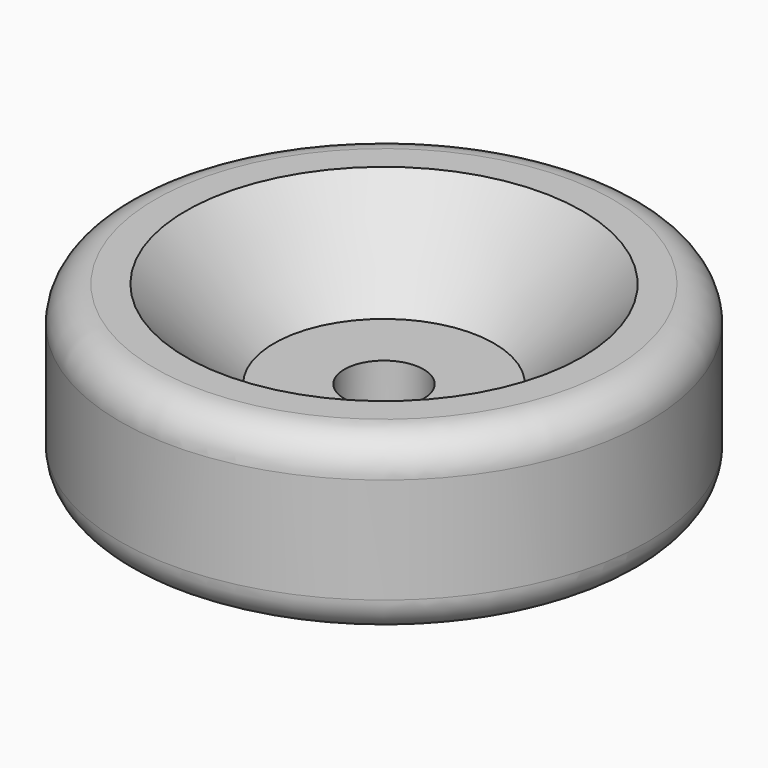
from build123d import *

# Parameters (mm, degrees)
F0_R     = 15
F0_R_2   = 11
F0_R_3   = 4.25
F1_DEPTH = 10
F2_R     = 2
F0_R_4   = 2.25
F3_DEPTH = 5


# Not quite as in the source:
# - a fillet or chamfer that OpenCascade refuses, or shapes differently, is made with other operations: its cross-section is extruded or revolved along the edge and cut away or added


with BuildPart() as f1:
    # F0 (on Top) → F1 (new body)
    with BuildSketch(Plane.XY):
        Circle(F0_R)
        Circle(F0_R_2, mode=Mode.SUBTRACT)
        Circle(F0_R_2)
        Circle(F0_R_3, mode=Mode.SUBTRACT)
    extrude(amount=F1_DEPTH)

    # F2
    f2_edges = [f1.edges().sort_by_distance(p)[0] for p in [
        (-15, 0, 10),
        (15, 0, 5),
        (-15, 0, 0),
    ]]
    fillet(f2_edges, radius=F2_R)

    # F0 (on Top) → F3 (join)
    with BuildSketch(Plane.XY):
        Circle(F0_R_3)
        Circle(F0_R_4, mode=Mode.SUBTRACT)
    extrude(amount=F3_DEPTH)

    # F4: chamfer of 7 on 1 edges, made by hand


with BuildPart() as f4_tool2:
    # F4_s3 → F4_t4 (revolve)
    with BuildSketch(Plane.XZ):
        Polygon((11.25, 10), (4.25, 3), (4.25, 10), align=None)
    revolve(axis=Axis((0, 0, 10), (0, 0, 1)))

    split(bisect_by=Plane.XY.offset(5), keep=Keep.TOP)


with BuildPart() as f1_1:
    add(f1.part)

    # F4_t1: cut F4_tool2
    add(f4_tool2.part, mode=Mode.SUBTRACT)


solid = f1_1.part
